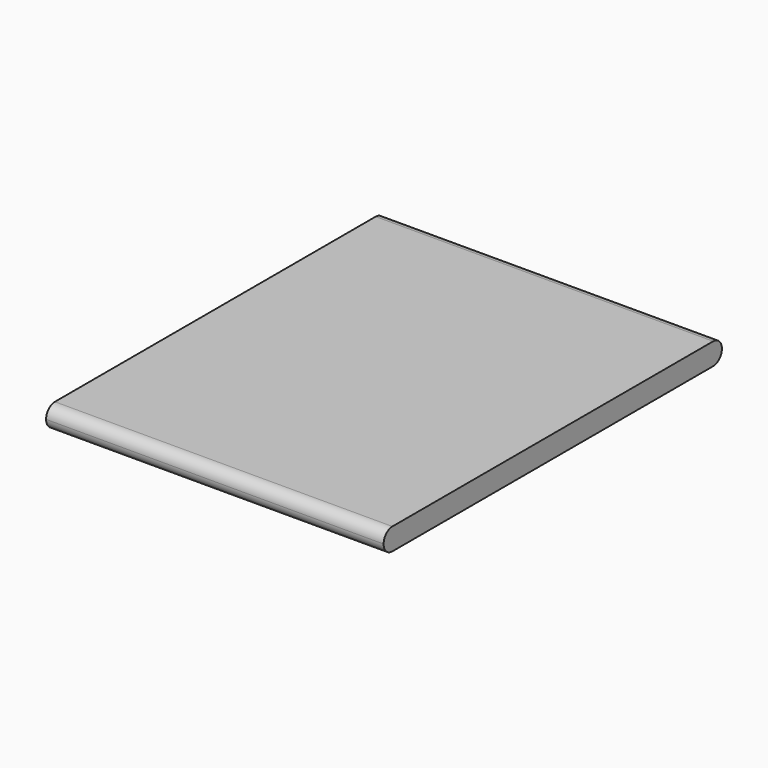
from build123d import *

# Parameters (mm, degrees)
F0_W     = 540
F0_H     = 28
F1_DEPTH = 431
F2_R     = 13.99999


# Not quite as in the source:
# - a fillet or chamfer is up to 0.001 mm smaller than in the source, because OpenCascade refuses the exact size


with BuildPart() as f1:
    # F0 (on Right) → F1 (new body)
    with BuildSketch(Plane.YZ):
        with Locations((202.4743151665, -5.4919481874)):
            Rectangle(F0_W, F0_H)
    extrude(amount=F1_DEPTH)

    # F2 (radius 14 in the source; OpenCascade refuses exactly that, so slightly less here)
    f2_edges = [f1.edges().sort_by_distance(p)[0] for p in [
        (215.5, -67.525685, 8.508052),
        (215.5, -67.525685, -19.491948),
        (215.5, 472.474315, 8.508052),
        (215.5, 472.474315, -19.491948),
    ]]
    fillet(f2_edges, radius=F2_R)


solid = f1.part
